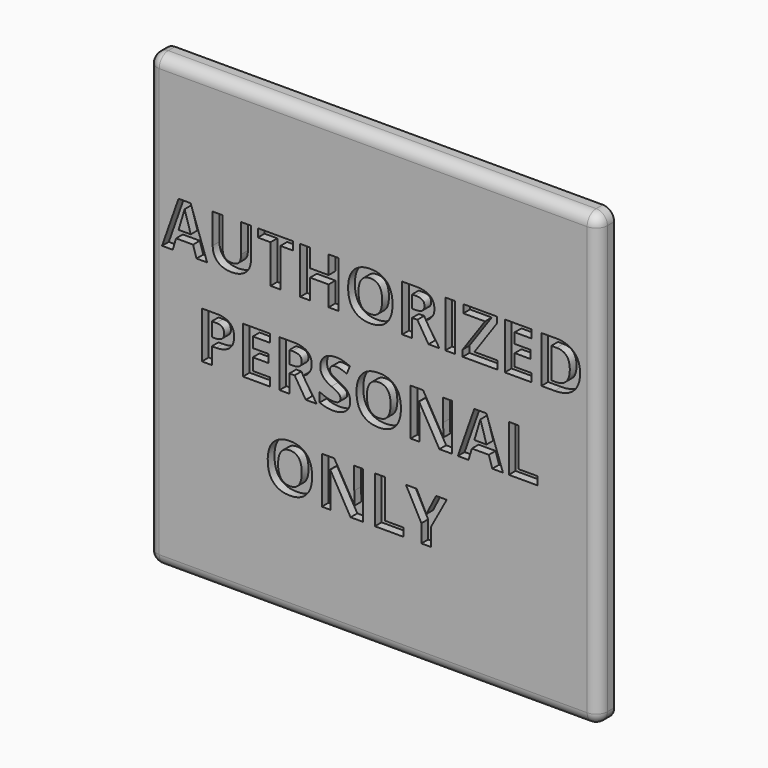
from build123d import *

# Parameters (mm, degrees)
F0_W         = 203.2
F0_H         = 203.2
F1_DEPTH     = 8.89
F3_R         = 5.08
F4_R         = 5.08
F5_R         = 5.08
F6_R         = 5.08
F7_R         = 5.08
F2_TEXT_SIZE = 29.4734806363
F8_DEPTH     = 3.81


# Not quite as in the source:
# - Text() gives the source's letters only with a copy of the font that has no kerning and outlines rounded to 1/6400 em; it was checked with that copy


with BuildPart() as f1:
    # F0 (on Front) → F1 (new body)
    with BuildSketch(Plane.XZ):
        Rectangle(F0_W, F0_H)
    extrude(amount=F1_DEPTH)

    # F3
    f3_edges = [f1.edges().sort_by_distance(p)[0] for p in [
        (101.6, -4.445, 101.6),
    ]]
    fillet(f3_edges, radius=F3_R)

    # F4
    f4_edges = [f1.edges().sort_by_distance(p)[0] for p in [
        (-101.6, -4.445, 101.6),
    ]]
    fillet(f4_edges, radius=F4_R)

    # F5
    f5_edges = [f1.edges().sort_by_distance(p)[0] for p in [
        (-101.6, -4.445, -101.6),
    ]]
    fillet(f5_edges, radius=F5_R)

    # F6
    f6_edges = [f1.edges().sort_by_distance(p)[0] for p in [
        (101.6, -4.445, -101.6),
    ]]
    fillet(f6_edges, radius=F6_R)

    # F7
    f7_edges = [f1.edges().sort_by_distance(p)[0] for p in [
        (0, -8.89, -101.6),
    ]]
    fillet(f7_edges, radius=F7_R)

    # F2 (on face) → F8 (cut)
    with BuildSketch(Plane.XZ.offset(8.89)):
        with Locations((-95.25, 26.5635480569)):
            Text('AUTHORIZED', F2_TEXT_SIZE, font='Open Sans', font_style=FontStyle.BOLD, text_align=(TextAlign.LEFT, TextAlign.BOTTOM))
        with Locations((-79.9330005318, -13.5203856084)):
            Text('PERSONAL', F2_TEXT_SIZE, font='Open Sans', font_style=FontStyle.BOLD, text_align=(TextAlign.LEFT, TextAlign.BOTTOM))
        with Locations((-49.2990015955, -53.6043192737)):
            Text('ONLY', F2_TEXT_SIZE, font='Open Sans', font_style=FontStyle.BOLD, text_align=(TextAlign.LEFT, TextAlign.BOTTOM))
    extrude(amount=-F8_DEPTH, mode=Mode.SUBTRACT)


solid = f1.part
